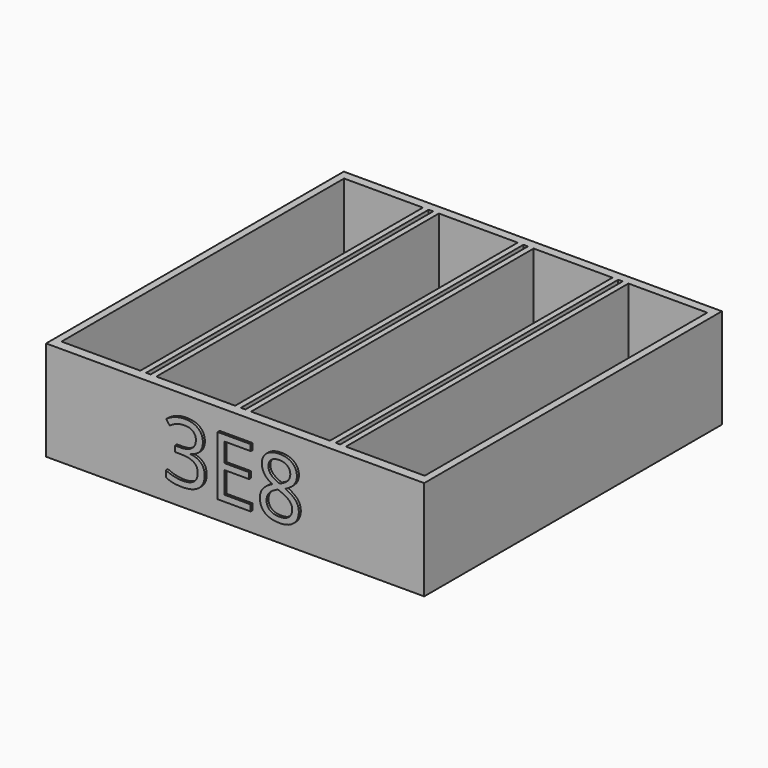
from build123d import *

# Parameters (mm, degrees)
F0_W         = 75.8
F0_H         = 74.6
F0_W_2       = 15.8
F0_H_2       = 70.8
F0_W_3       = 0.9
F1_DEPTH     = 20
F2_TEXT_SIZE = 16.6311218507
F3_DEPTH     = 0.5


# Not quite as in the source:
# - Text() gives the source's letters only with a copy of the font that has no kerning and outlines rounded to 1/6400 em; it was checked with that copy


with BuildPart() as f1:
    # F0 (on Top) → F1 (new body)
    with BuildSketch(Plane.XY):
        with Locations((28.5, -0.1)):
            Rectangle(F0_W, F0_H)
        Rectangle(F0_W_2, F0_H_2, mode=Mode.SUBTRACT)
        with Locations((9.5, 0)):
            Rectangle(F0_W_3, F0_H_2, mode=Mode.SUBTRACT)
        with Locations((19, 0)):
            Rectangle(F0_W_2, F0_H_2, mode=Mode.SUBTRACT)
        with Locations((28.5, 0)):
            Rectangle(F0_W_3, F0_H_2, mode=Mode.SUBTRACT)
        with Locations((38, 0)):
            Rectangle(F0_W_2, F0_H_2, mode=Mode.SUBTRACT)
        with Locations((47.5, 0)):
            Rectangle(F0_W_3, F0_H_2, mode=Mode.SUBTRACT)
        with Locations((57, 0)):
            Rectangle(F0_W_2, F0_H_2, mode=Mode.SUBTRACT)
    extrude(amount=F1_DEPTH)

    # F2 (on face) → F3 (join)
    with BuildSketch(Plane.XZ.offset(37.4)):
        with Locations((14.258302609, 4.0127961338)):
            Text('3E8', F2_TEXT_SIZE, font='Open Sans', text_align=(TextAlign.LEFT, TextAlign.BOTTOM))
    extrude(amount=F3_DEPTH)


solid = f1.part
